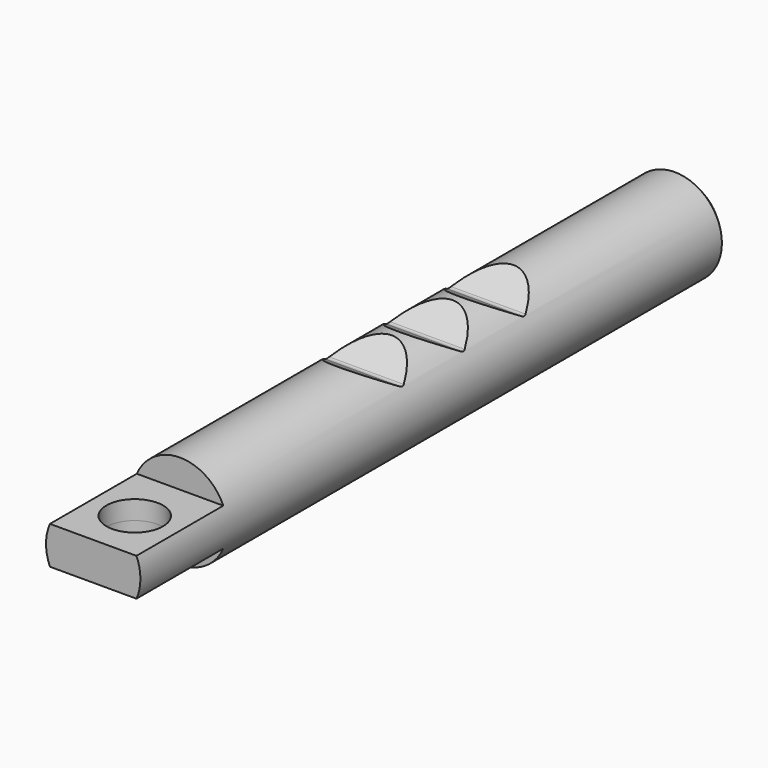
from build123d import *

# Parameters (mm, degrees)
F0_R          = 10
F1_DEPTH      = 156
F2_SIZE       = 2
F3_W          = 20
F3_H          = 8
F4_DEPTH      = 23
F5_R          = 6
F6_DEPTH      = 10.001
F6_DEPTH_BACK = 10.001
F8_DEPTH      = 10.001
F8_DEPTH_BACK = 10.001


# Not quite as in the source:
# - a pattern or mirror of a feature is missing from the dataset's text; its kind, count and spacing are read off the source's solid


with BuildPart() as f1:
    # F0 (on Front) → F1 (new body)
    with BuildSketch(Plane.XZ):
        Circle(F0_R)
    extrude(amount=-F1_DEPTH)

    # F2
    f2_edges = [f1.edges().sort_by_distance(p)[0] for p in [
        (-10, 156, 0),
    ]]
    chamfer(f2_edges, length=F2_SIZE)

    # F3 (on Front) → F4 (cut)
    with BuildSketch(Plane.XZ):
        with Locations((0, 8)):
            Rectangle(F3_W, F3_H)
    f4 = extrude(amount=-F4_DEPTH, mode=Mode.SUBTRACT)

    # F4_copies: F4 across plane
    add(f4.mirror(Plane(origin=(0, 0, 0), x_dir=(-1, 0, 0), z_dir=(0, 0, -1))), mode=Mode.SUBTRACT)

    # F5 (on Top) → F6 (cut, two sides)
    with BuildSketch(Plane.XY) as f6_sk:
        with Locations((0, 11)):
            Circle(F5_R)
    extrude(amount=-F6_DEPTH, mode=Mode.SUBTRACT)
    extrude(f6_sk.sketch, amount=F6_DEPTH_BACK, mode=Mode.SUBTRACT)

    # F7 (on Right) → F8 (cut, two sides)
    with BuildSketch(Plane.YZ) as f8_sk:
        with BuildLine():
            Line((96.0621778265, 10.5), (79.9378221735, 10.5))
            Line((79.9378221735, 10.5), (87.5, 6.1339745962))
            ThreePointArc((87.5, 6.1339745962), (88, 6), (88.5, 6.1339745962))
            Line((88.5, 6.1339745962), (96.0621778265, 10.5))
        make_face()
        with BuildLine():
            Line((112.1865334795, 10.5), (96.0621778265, 10.5))
            Line((96.0621778265, 10.5), (103.624355653, 6.1339745962))
            ThreePointArc((103.624355653, 6.1339745962), (104.124355653, 6), (104.624355653, 6.1339745962))
            Line((104.624355653, 6.1339745962), (112.1865334795, 10.5))
        make_face()
        with BuildLine():
            Line((72.375644347, 6.1339745962), (79.9378221735, 10.5))
            Line((79.9378221735, 10.5), (63.8134665205, 10.5))
            Line((63.8134665205, 10.5), (71.375644347, 6.1339745962))
            ThreePointArc((71.375644347, 6.1339745962), (71.875644347, 6), (72.375644347, 6.1339745962))
        make_face()
    extrude(amount=-F8_DEPTH, mode=Mode.SUBTRACT)
    extrude(f8_sk.sketch, amount=F8_DEPTH_BACK, mode=Mode.SUBTRACT)


solid = f1.part
